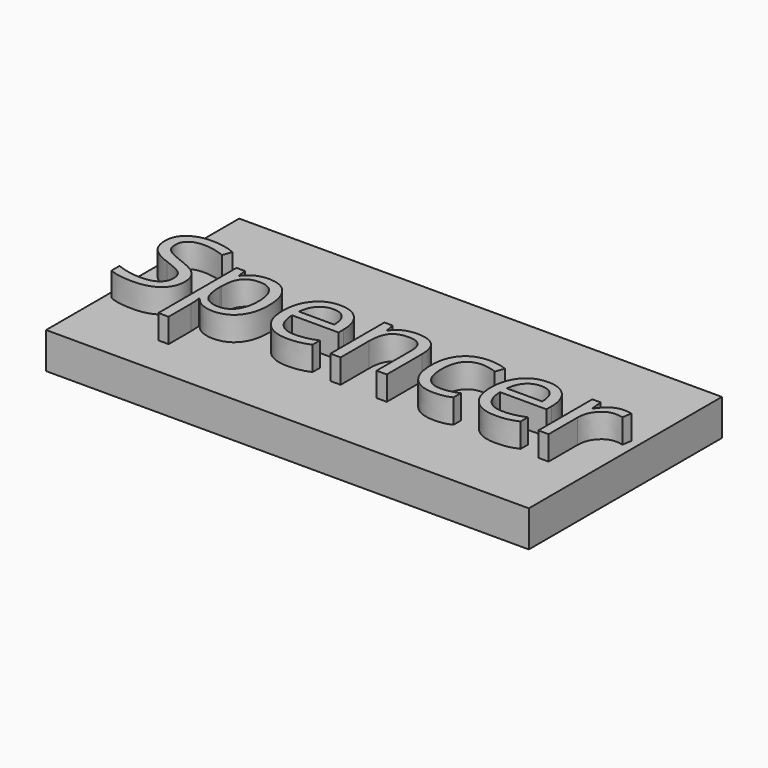
from build123d import *

# Parameters (mm, degrees)
F0_W         = 40
F0_H         = 20
F1_DEPTH     = 3
F2_TEXT_SIZE = 10.4366260345
F3_DEPTH     = 5


# Not quite as in the source:
# - Text() gives the source's letters only with a copy of the font that has no kerning and outlines rounded to 1/6400 em; it was checked with that copy


with BuildPart() as f1:
    # F0 (on Top) → F1 (new body)
    with BuildSketch(Plane.XY):
        with Locations((23.9408151247, 12.8827810279)):
            Rectangle(F0_W, F0_H)
    extrude(amount=F1_DEPTH)

    # F2 (on Top) → F3 (join)
    with BuildSketch(Plane.XY):
        with Locations((3.8977924717, 8.7925686141)):
            Text('Spencer', F2_TEXT_SIZE, font='Open Sans', text_align=(TextAlign.LEFT, TextAlign.BOTTOM))
    extrude(amount=F3_DEPTH)


solid = f1.part
